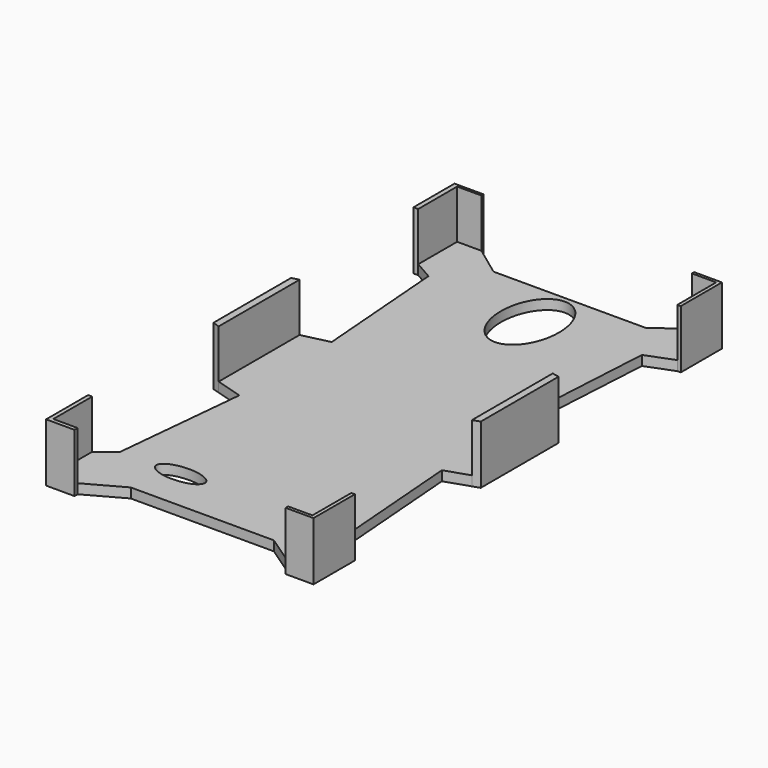
from build123d import *

# Parameters (mm, degrees)
F0_W     = 69.85
F0_H     = 133.35
F1_DEPTH = 15.24
F3_DEPTH = 15.241
F4_DEPTH = 15.241
F5_DEPTH = 12.7
F6_DEPTH = 15.2410001


# Not quite as in the source:
# - a feature names something its author has since deleted; it is built from what else it names


with BuildPart() as f1:
    # F0 (on Top) → F1 (new body)
    with BuildSketch(Plane.XY):
        with Locations((-4.9132461604, -3.2689645886)):
            Rectangle(F0_W, F0_H)
    extrude(amount=F1_DEPTH)

    # F2 (on face) → F3 (cut, through all)
    with BuildSketch(Plane.XY.offset(15.24)):
        Polygon((-4.9132461604, 63.4060354114), (-32.2555484414, 63.4060354114), (-32.2555484414, 62.717136082), (-24.5693009347, 57.0560354114), (-4.9132461604, 57.0560354114), align=None)
        Polygon((-38.6055484414, 50.017136082), (-39.8382461604, 50.017136082), (-39.8382461604, 10.0660354114), (-37.9972373044, 10.4986778455), (-30.9245064855, 12.1607901528), (-33.6875207722, 47.2298189998), align=None)
        Polygon((22.7516740561, 63.4060354114), (-4.9132461604, 63.4060354114), (-4.9132461604, 57.0560354114), (15.2570633218, 57.0560354114), (22.7516740561, 62.6652065337), align=None)
        Polygon((-37.9972373044, -15.8886924859), (-39.8382461604, -15.3339645886), (-39.8382461604, -55.9739645886), (-39.8382461604, -56.2118504524), (-38.7796634255, -56.2118504524), (-34.3251377344, -52.876316011), (-30.9245064855, -18.0198289454), align=None)
        Polygon((30.0117538396, 49.9652065337), (29.1016740561, 49.9652065337), (22.0408134996, 47.2298189998), (20.0073712407, 12.1607901528), (28.1864475644, 10.4482248105), (30.0117538396, 10.0660354114), align=None)
        Polygon((-32.4296634255, -68.9118504524), (-32.4296634255, -69.9439645886), (-6.858468987, -69.9439645886), (-6.858468987, -63.5939645886), (-22.7989349514, -63.5939645886), align=None)
        Polygon((30.0117538396, -55.9739645886), (30.0117538396, -15.3339645886), (28.1864475644, -15.9457166114), (21.9978448004, -18.0198289454), (24.7441133717, -52.876316011), (29.0817226684, -56.4274404526), (30.0117538396, -56.4274404526), align=None)
        Polygon((-6.858468987, -63.5939645886), (-6.858468987, -69.9439645886), (22.7317226684, -69.9439645886), (22.7317226684, -69.1274404526), (14.6080274135, -63.5939645886), align=None)
    extrude(amount=-F3_DEPTH, mode=Mode.SUBTRACT)

    # F2 (on face) → F4 (cut, through all)
    with BuildSketch(Plane.XY.offset(15.24)):
        with BuildLine():
            add(Edge.make_bspline(
                [(-4.9132461604, 32.9410274994), (8.2097492076, 32.9410274994), (1.6482515236, 50.0860274994), (-4.9132461604, 67.2310274994), (-11.4747438444, 50.0860274994), (-18.0362415283, 32.9410274994), (-4.9132461604, 32.9410274994)],
                knots=[0, 0, 0, 2.0943951024, 2.0943951024, 4.1887902048, 4.1887902048, 6.2831853072, 6.2831853072, 6.2831853072], degree=2, weights=[1, 0.5, 1, 0.5, 1, 0.5, 1]))
        make_face()
    extrude(amount=-F4_DEPTH, mode=Mode.SUBTRACT)

    # F2 (on face) → F5 (cut)
    with BuildSketch(Plane.XY.offset(15.24)):
        Polygon((-24.5693009347, 57.0560354114), (-32.2555484414, 62.717136082), (-38.6055484414, 62.717136082), (-38.6055484414, 50.017136082), (-33.6875207722, 47.2298189998), (-30.9245064855, 12.1607901528), (-37.9972373044, 10.4986778455), (-37.9972373044, -15.8886924859), (-30.9245064855, -18.0198289454), (-34.3251377344, -52.876316011), (-38.7796634255, -56.2118504524), (-38.7796634255, -68.9118504524), (-32.4296634255, -68.9118504524), (-22.7989349514, -63.5939645886), (-6.858468987, -63.5939645886), (14.6080274135, -63.5939645886), (22.7317226684, -69.1274404526), (29.0817226684, -69.1274404526), (29.0817226684, -56.4274404526), (24.7441133717, -52.876316011), (21.9978448004, -18.0198289454), (28.1864475644, -15.9457166114), (28.1864475644, 10.4482248105), (20.0073712407, 12.1607901528), (22.0408134996, 47.2298189998), (29.1016740561, 49.9652065337), (29.1016740561, 62.6652065337), (22.7516740561, 62.6652065337), (15.2570633218, 57.0560354114), (-4.9132461604, 57.0560354114), align=None)
        with BuildLine():
            add(Edge.make_bspline(
                [(-12.2060639948, -52.6248924434), (-12.2060639948, -47.7662279623), (-21.7310639948, -50.1955602028), (-31.2560639948, -52.6248924434), (-21.7310639948, -55.054224684), (-12.2060639948, -57.4835569246), (-12.2060639948, -52.6248924434)],
                knots=[0, 0, 0, 2.0943951024, 2.0943951024, 4.1887902048, 4.1887902048, 6.2831853072, 6.2831853072, 6.2831853072], degree=2, weights=[1, 0.5, 1, 0.5, 1, 0.5, 1]))
        make_face(mode=Mode.SUBTRACT)
        with BuildLine():
            add(Edge.make_bspline(
                [(-4.9132461604, 32.9410274994), (8.2097492076, 32.9410274994), (1.6482515236, 50.0860274994), (-4.9132461604, 67.2310274994), (-11.4747438444, 50.0860274994), (-18.0362415283, 32.9410274994), (-4.9132461604, 32.9410274994)],
                knots=[0, 0, 0, 2.0943951024, 2.0943951024, 4.1887902048, 4.1887902048, 6.2831853072, 6.2831853072, 6.2831853072], degree=2, weights=[1, 0.5, 1, 0.5, 1, 0.5, 1]))
        make_face(mode=Mode.SUBTRACT)
    extrude(amount=-F5_DEPTH, mode=Mode.SUBTRACT)

    # F6 (cut, through all): a face of the model
    f6_faces = [f1.faces().sort_by_distance(p)[0] for p in [
        (-18.5223410281, -52.6248924434, 15.24),
    ]]
    extrude(f6_faces, amount=-F6_DEPTH, mode=Mode.SUBTRACT)


solid = f1.part
